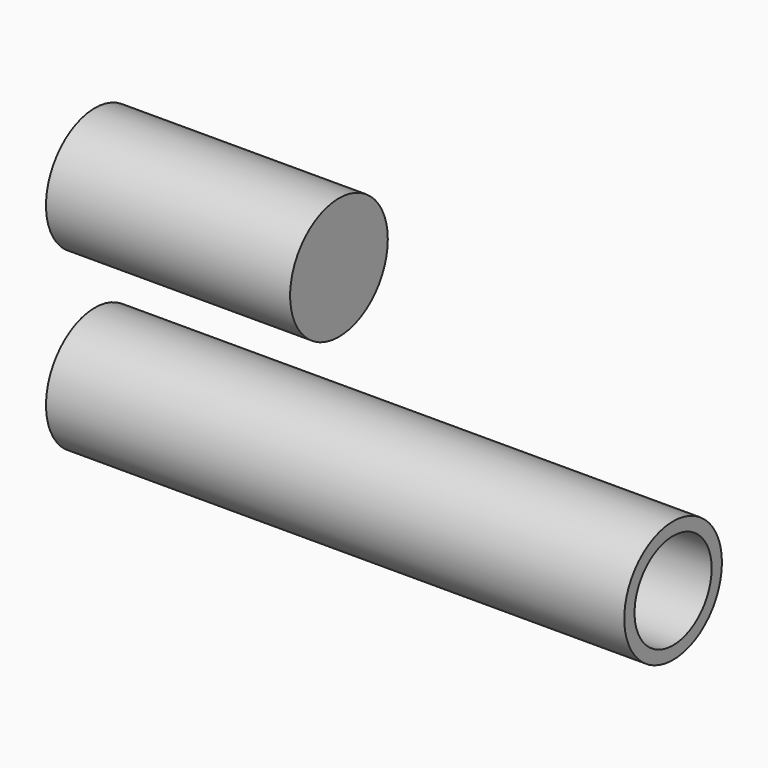
from build123d import *

# Parameters (mm, degrees)
F0_R      = 4.75
F0_R_2    = 3.75
F1_DEPTH  = 45
F2_R      = 4.75
F3_DEPTH  = 19
F3_FACE_R = 4.75


# Not quite as in the source:
# - an extrude whose draft closes it to a point is written as a loft to that point


with BuildPart() as f1:
    # F0 (on Right) → F1 (new body)
    with BuildSketch(Plane.YZ):
        Circle(F0_R)
        Circle(F0_R_2, mode=Mode.SUBTRACT)
    extrude(amount=F1_DEPTH)


with BuildPart() as f3:
    # F2 (on Right) → F3 (new body)
    with BuildSketch(Plane.YZ):
        with Locations((0, 13.678194955)):
            Circle(F2_R)
    extrude(amount=F3_DEPTH)

    # F3_face (on face) → F4 section 0
    with BuildSketch(Plane(origin=(0, 0, 13.678194955), x_dir=(0, 1, 0), z_dir=(-1, 0, 0)), mode=Mode.PRIVATE) as f4_s0:
        Circle(F3_FACE_R)
    loft([f4_s0.sketch, Vertex(19.0512094343, 0, 13.678194955)], ruled=True, mode=Mode.SUBTRACT)


solid = Compound([f1.part, f3.part])
